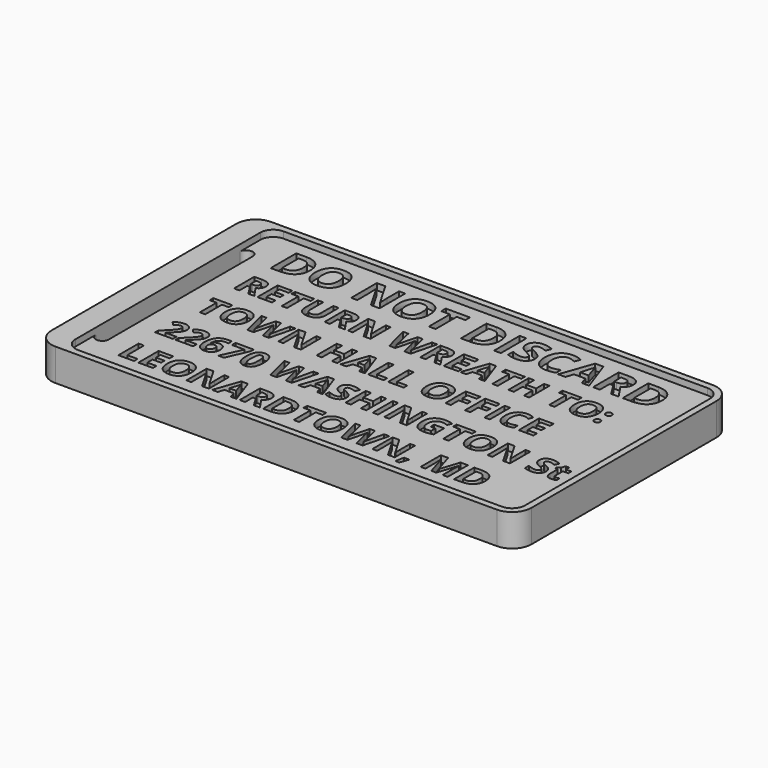
from build123d import *

# Parameters (mm, degrees)
F1_DEPTH       = 6.35
F2_DEPTH       = 5.08
F3_TEXT_SIZE   = 8.8599821957
F3_TEXT_SIZE_2 = 7.0061295972
F4_DEPTH       = 1.27


# Not quite as in the source:
# - Text() gives the source's letters only with a copy of the font that has no kerning and outlines rounded to 1/6400 em; it was checked with that copy


with BuildPart() as f1:
    # F0 (on Top) → F1 (new body)
    with BuildSketch(Plane.XY):
        with BuildLine():
            Line((-0.9129742631, -1.27), (2.8970257369, -1.27))
            Line((2.8970257369, -1.27), (86.36, -1.27))
            ThreePointArc((86.36, -1.27), (89.0540768363, -0.1540768363), (90.17, 2.54))
            Line((90.17, 2.54), (90.17, 48.26))
            ThreePointArc((90.17, 48.26), (89.1835421071, 50.8360700741), (86.7170257369, 52.0711948439))
            Line((86.7170257369, 52.0711948439), (2.8970257369, 52.0711948439))
            Line((2.8970257369, 52.0711948439), (-0.9129742631, 52.0711948439))
            ThreePointArc((-0.9129742631, 52.0711948439), (-3.6070510995, 50.9552716802), (-4.7229742631, 48.2611948439))
            Line((-4.7229742631, 48.2611948439), (-4.7229742631, 2.54))
            ThreePointArc((-4.7229742631, 2.54), (-3.6070510995, -0.1540768363), (-0.9129742631, -1.27))
        make_face()
        with BuildLine():
            Line((86.36, 0), (2.54, 0))
            ThreePointArc((2.54, 0), (0.7439487758, 0.7439487758), (0, 2.54))
            Line((0, 2.54), (0, 7.62))
            Line((0, 7.62), (0, 43.18))
            Line((0, 43.18), (0, 48.26))
            ThreePointArc((0, 48.26), (0.7439487758, 50.0560512242), (2.54, 50.8))
            Line((2.54, 50.8), (86.36, 50.8))
            ThreePointArc((86.36, 50.8), (88.1560512242, 50.0560512242), (88.9, 48.26))
            Line((88.9, 48.26), (88.9, 2.54))
            ThreePointArc((88.9, 2.54), (88.1560512242, 0.7439487758), (86.36, 0))
        make_face(mode=Mode.SUBTRACT)
    extrude(amount=F1_DEPTH)

    # F0 (on Top) → F2 (join)
    with BuildSketch(Plane.XY):
        with BuildLine():
            ThreePointArc((0, 2.54), (0.7439487758, 0.7439487758), (2.54, 0))
            Line((2.54, 0), (86.36, 0))
            ThreePointArc((86.36, 0), (88.1560512242, 0.7439487758), (88.9, 2.54))
            Line((88.9, 2.54), (88.9, 48.26))
            ThreePointArc((88.9, 48.26), (88.1560512242, 50.0560512242), (86.36, 50.8))
            Line((86.36, 50.8), (2.54, 50.8))
            ThreePointArc((2.54, 50.8), (0.7439487758, 50.0560512242), (0, 48.26))
            Line((0, 48.26), (0, 43.18))
            ThreePointArc((0, 43.18), (1.27, 44.45), (2.54, 43.18))
            Line((2.54, 43.18), (2.54, 25.4))
            Line((2.54, 25.4), (2.54, 7.62))
            ThreePointArc((2.54, 7.62), (1.27, 6.35), (0, 7.62))
            Line((0, 7.62), (0, 2.54))
        make_face()
    extrude(amount=F2_DEPTH)

    # F3 (on face) → F4 (cut)
    with BuildSketch(Plane.XY.offset(5.08)):
        with Locations((6.35, 41.8808128191)):
            Text('DO NOT DISCARD', F3_TEXT_SIZE, font='Open Sans', font_style=FontStyle.BOLD, text_align=(TextAlign.LEFT, TextAlign.BOTTOM))
        with Locations((6.35, 33.0263995091)):
            Text('RETURN WREATH TO:', F3_TEXT_SIZE_2, font='Open Sans', font_style=FontStyle.BOLD, text_align=(TextAlign.LEFT, TextAlign.BOTTOM))
        with Locations((6.35, 23.4980632569)):
            Text('TOWN HALL OFFICE', F3_TEXT_SIZE_2, font='Open Sans', font_style=FontStyle.BOLD, text_align=(TextAlign.LEFT, TextAlign.BOTTOM))
        with Locations((6.35, 13.9697270047)):
            Text('22670 WASHINGTON St', F3_TEXT_SIZE_2, font='Open Sans', font_style=FontStyle.BOLD, text_align=(TextAlign.LEFT, TextAlign.BOTTOM))
        with Locations((6.35, 4.4413907525)):
            Text('LEONARDTOWN, MD', F3_TEXT_SIZE_2, font='Open Sans', font_style=FontStyle.BOLD, text_align=(TextAlign.LEFT, TextAlign.BOTTOM))
    extrude(amount=-F4_DEPTH, mode=Mode.SUBTRACT)


solid = f1.part
